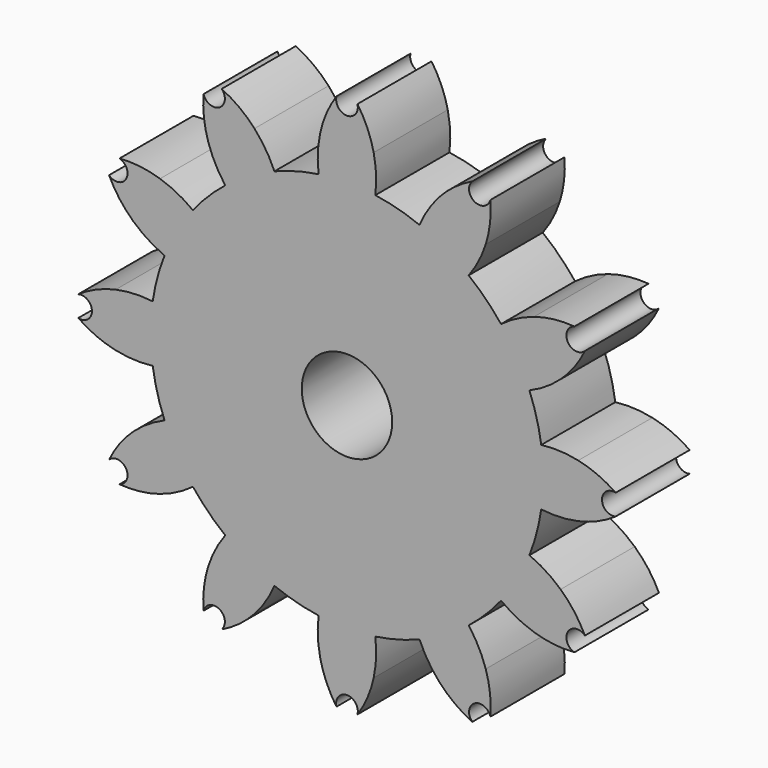
from build123d import *

# Parameters (mm, degrees)
F1_DEPTH = 12.6
F2_COUNT = 12
F3_R     = 6.1544610685
F4_DEPTH = 25


with BuildPart() as f1:
    # F0 (on Front) → F1 (new body)
    with BuildSketch(Plane.XZ):
        with BuildLine():
            ThreePointArc((2.7852032442, 25.3538235305), (-10.8298302985, -21.3004259569), (33.3673953593, -1.0867331287))
            ThreePointArc((33.3673953593, -1.0867331287), (26.8600881876, 16.3894925292), (10.5075874745, 25.3538235305))
            ThreePointArc((10.5075874745, 25.3538235305), (8.9226743944, 25.5371357629), (7.3296460588, 25.6255301502))
            ThreePointArc((7.3296460588, 25.6255301502), (5.0516276545, 25.5866348058), (2.7852032442, 25.3538235305))
        make_face()
        with BuildLine():
            ThreePointArc((7.3296460588, 25.6255301502), (8.9226743944, 25.5371357629), (10.5075874745, 25.3538235305))
            ThreePointArc((10.5075874745, 25.3538235305), (10.6097622585, 27.8798441888), (10.28181369, 30.3865691018))
            ThreePointArc((10.28181369, 30.3865691018), (9.4245102455, 33.0410725411), (8.0713397316, 35.4803936077))
            ThreePointArc((8.0713397316, 35.4803936077), (6.6463953593, 33.6211668014), (5.2214509871, 35.4803936077))
            ThreePointArc((5.2214509871, 35.4803936077), (3.8682804732, 33.0410725411), (3.0109770287, 30.3865691018))
            ThreePointArc((3.0109770287, 30.3865691018), (2.6830284602, 27.8798441888), (2.7852032442, 25.3538235305))
            ThreePointArc((2.7852032442, 25.3538235305), (5.0516276545, 25.5866348058), (7.3296460588, 25.6255301502))
        make_face()
    extrude(amount=F1_DEPTH)

    # F2: F1 ×12 about axis
    f2_axis = Axis((6.6463953593, 0, -1.0867331287), (0, 1, 0))


with BuildPart() as f1_1:
    add(f1.part)
    for i in range(1, F2_COUNT):
        add(f1.part.rotate(f2_axis, i * 360 / F2_COUNT))

    # F3 (on face) → F4 (cut)
    with BuildSketch(Plane.XZ.offset(12.6)):
        with Locations((6.6463953593, -1.0867331287)):
            Circle(F3_R)
    extrude(amount=-F4_DEPTH, mode=Mode.SUBTRACT)


solid = f1_1.part
